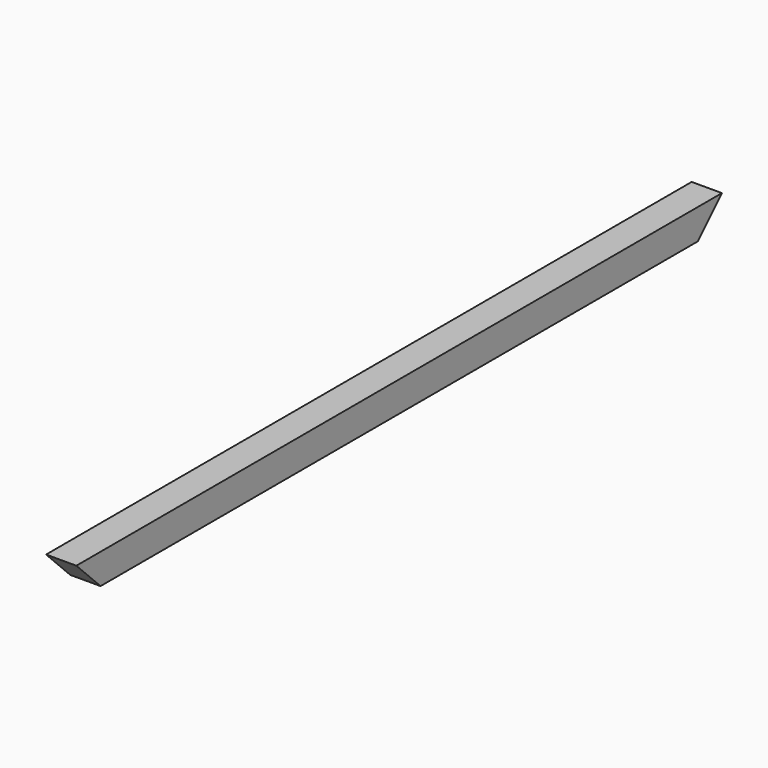
from build123d import *

# Parameters (mm, degrees)
F0_W     = 3.81
F0_H     = 101.6
F1_DEPTH = 3.81
F2_SIZE  = 3.80999
F3_SIZE  = 3.80999


# Not quite as in the source:
# - a fillet or chamfer is up to 0.001 mm smaller than in the source, because OpenCascade refuses the exact size


with BuildPart() as f1:
    # F0 (on Top) → F1 (new body)
    with BuildSketch(Plane.XY):
        with Locations((49.9639250338, 45.283157554)):
            Rectangle(F0_W, F0_H)
    extrude(amount=F1_DEPTH)

    # F2 (size 3.81 in the source; OpenCascade refuses exactly that, so slightly less here)
    f2_edges = [f1.edges().sort_by_distance(p)[0] for p in [
        (49.963925, -5.516842, 0),
    ]]
    chamfer(f2_edges, length=F2_SIZE)

    # F3 (size 3.81 in the source; OpenCascade refuses exactly that, so slightly less here)
    f3_edges = [f1.edges().sort_by_distance(p)[0] for p in [
        (49.963925, 96.083158, 0),
    ]]
    chamfer(f3_edges, length=F3_SIZE)


solid = f1.part
